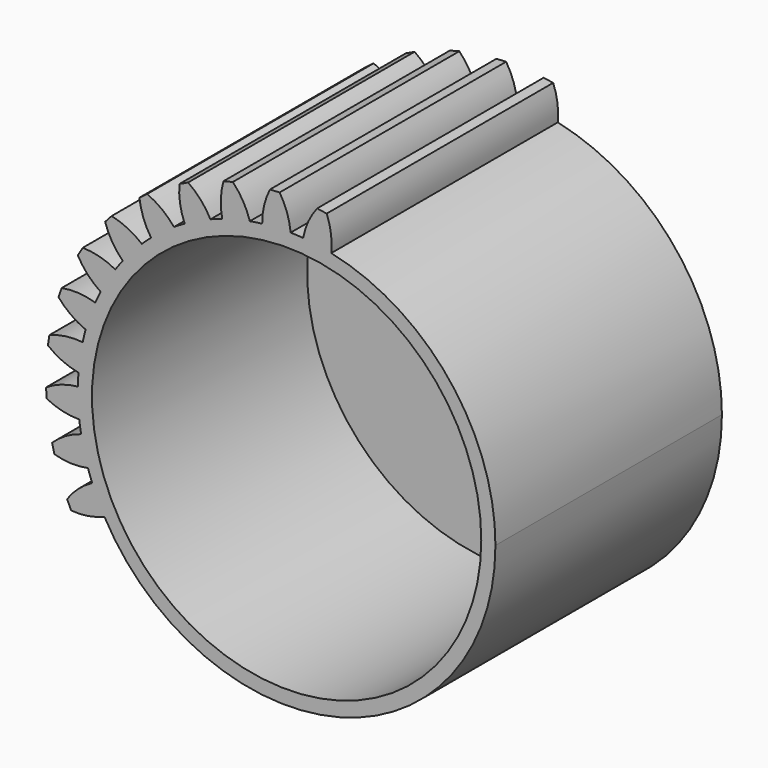
from build123d import *

# Parameters (mm, degrees)
F0_R     = 55
F1_DEPTH = 80
F2_DEPTH = 80
F3_DEPTH = 4


with BuildPart() as f1:
    # F0 (on Front) → F1 (new body)
    with BuildSketch(Plane.XZ):
        with BuildLine():
            ThreePointArc((-51.4911909934, -28.8037714558), (14.8832075069, -57.0919445658), (59, 0))
            ThreePointArc((59, 0), (45.9639360321, 36.9907635016), (12.6163869683, 57.6352910973))
            ThreePointArc((12.6163869683, 57.6352910973), (8.6570979929, 58.3614140879), (4.6575122934, 58.8158786319))
            ThreePointArc((4.6575122934, 58.8158786319), (2.8949927853, 58.9289319161), (1.1298791308, 58.9891801363))
            ThreePointArc((1.1298791308, 58.9891801363), (-2.8949927853, 58.9289319161), (-6.9063892013, 58.5943835892))
            ThreePointArc((-6.9063892013, 58.5943835892), (-8.6570979929, 58.3614140879), (-10.4000493282, 58.0761480642))
            ThreePointArc((-10.4000493282, 58.0761480642), (-14.3358306143, 57.2318439385), (-18.2048820321, 56.1211392454))
            ThreePointArc((-18.2048820321, 56.1211392454), (-19.8765013501, 55.5510998458), (-21.5303097238, 54.9312821914))
            ThreePointArc((-21.5303097238, 54.9312821914), (-25.2257505124, 53.3353682943), (-28.8037714558, 51.4911909934))
            ThreePointArc((-28.8037714558, 51.4911909934), (-30.3320619074, 50.60598799), (-31.8331723911, 49.6754379499))
            ThreePointArc((-31.8331723911, 49.6754379499), (-35.1462589651, 47.3892443574), (-38.2957480959, 44.8824651482))
            ThreePointArc((-38.2957480959, 44.8824651482), (-39.621978336, 43.7161163959), (-40.9127040957, 42.5105944863))
            ThreePointArc((-40.9127040957, 42.5105944863), (-43.7161163959, 39.621978336), (-46.3160406131, 36.5489313377))
            ThreePointArc((-46.3160406131, 36.5489313377), (-47.3892443574, 35.1462589651), (-48.419983526, 33.7120927168))
            ThreePointArc((-48.419983526, 33.7120927168), (-50.60598799, 30.3320619074), (-52.5564336639, 26.8108425927))
            ThreePointArc((-52.5564336639, 26.8108425927), (-53.3353682943, 25.2257505124), (-54.0665101436, 23.6180541301))
            ThreePointArc((-54.0665101436, 23.6180541301), (-55.5510998458, 19.8765013501), (-56.777112443, 16.0424282026))
            ThreePointArc((-56.777112443, 16.0424282026), (-57.2318439385, 14.3358306143), (-57.6352910973, 12.6163869683))
            ThreePointArc((-57.6352910973, 12.6163869683), (-58.3614140879, 8.6570979929), (-58.8158786319, 4.6575122934))
            ThreePointArc((-58.8158786319, 4.6575122934), (-58.9289319161, 2.8949927853), (-58.9891801363, 1.1298791308))
            ThreePointArc((-58.9891801363, 1.1298791308), (-58.9289319161, -2.8949927853), (-58.5943835892, -6.9063892013))
            ThreePointArc((-58.5943835892, -6.9063892013), (-58.3614140879, -8.6570979929), (-58.0761480642, -10.4000493282))
            ThreePointArc((-58.0761480642, -10.4000493282), (-57.2318439385, -14.3358306143), (-56.1211392454, -18.2048820321))
            ThreePointArc((-56.1211392454, -18.2048820321), (-55.5510998458, -19.8765013501), (-54.9312821914, -21.5303097238))
            ThreePointArc((-54.9312821914, -21.5303097238), (-53.3353682943, -25.2257505124), (-51.4911909934, -28.8037714558))
        make_face()
        Circle(F0_R, mode=Mode.SUBTRACT)
    extrude(amount=F1_DEPTH)

    # F0 (on Front) → F2 (join)
    with BuildSketch(Plane.XZ):
        with BuildLine():
            ThreePointArc((-51.4911909934, -28.8037714558), (14.8832075069, -57.0919445658), (59, 0))
            ThreePointArc((59, 0), (45.9639360321, 36.9907635016), (12.6163869683, 57.6352910973))
            ThreePointArc((12.6163869683, 57.6352910973), (8.6570979929, 58.3614140879), (4.6575122934, 58.8158786319))
            ThreePointArc((4.6575122934, 58.8158786319), (2.8949927853, 58.9289319161), (1.1298791308, 58.9891801363))
            ThreePointArc((1.1298791308, 58.9891801363), (-2.8949927853, 58.9289319161), (-6.9063892013, 58.5943835892))
            ThreePointArc((-6.9063892013, 58.5943835892), (-8.6570979929, 58.3614140879), (-10.4000493282, 58.0761480642))
            ThreePointArc((-10.4000493282, 58.0761480642), (-14.3358306143, 57.2318439385), (-18.2048820321, 56.1211392454))
            ThreePointArc((-18.2048820321, 56.1211392454), (-19.8765013501, 55.5510998458), (-21.5303097238, 54.9312821914))
            ThreePointArc((-21.5303097238, 54.9312821914), (-25.2257505124, 53.3353682943), (-28.8037714558, 51.4911909934))
            ThreePointArc((-28.8037714558, 51.4911909934), (-30.3320619074, 50.60598799), (-31.8331723911, 49.6754379499))
            ThreePointArc((-31.8331723911, 49.6754379499), (-35.1462589651, 47.3892443574), (-38.2957480959, 44.8824651482))
            ThreePointArc((-38.2957480959, 44.8824651482), (-39.621978336, 43.7161163959), (-40.9127040957, 42.5105944863))
            ThreePointArc((-40.9127040957, 42.5105944863), (-43.7161163959, 39.621978336), (-46.3160406131, 36.5489313377))
            ThreePointArc((-46.3160406131, 36.5489313377), (-47.3892443574, 35.1462589651), (-48.419983526, 33.7120927168))
            ThreePointArc((-48.419983526, 33.7120927168), (-50.60598799, 30.3320619074), (-52.5564336639, 26.8108425927))
            ThreePointArc((-52.5564336639, 26.8108425927), (-53.3353682943, 25.2257505124), (-54.0665101436, 23.6180541301))
            ThreePointArc((-54.0665101436, 23.6180541301), (-55.5510998458, 19.8765013501), (-56.777112443, 16.0424282026))
            ThreePointArc((-56.777112443, 16.0424282026), (-57.2318439385, 14.3358306143), (-57.6352910973, 12.6163869683))
            ThreePointArc((-57.6352910973, 12.6163869683), (-58.3614140879, 8.6570979929), (-58.8158786319, 4.6575122934))
            ThreePointArc((-58.8158786319, 4.6575122934), (-58.9289319161, 2.8949927853), (-58.9891801363, 1.1298791308))
            ThreePointArc((-58.9891801363, 1.1298791308), (-58.9289319161, -2.8949927853), (-58.5943835892, -6.9063892013))
            ThreePointArc((-58.5943835892, -6.9063892013), (-58.3614140879, -8.6570979929), (-58.0761480642, -10.4000493282))
            ThreePointArc((-58.0761480642, -10.4000493282), (-57.2318439385, -14.3358306143), (-56.1211392454, -18.2048820321))
            ThreePointArc((-56.1211392454, -18.2048820321), (-55.5510998458, -19.8765013501), (-54.9312821914, -21.5303097238))
            ThreePointArc((-54.9312821914, -21.5303097238), (-53.3353682943, -25.2257505124), (-51.4911909934, -28.8037714558))
        make_face()
        Circle(F0_R, mode=Mode.SUBTRACT)
        with BuildLine():
            ThreePointArc((4.6575122934, 58.8158786319), (8.6570979929, 58.3614140879), (12.6163869683, 57.6352910973))
            ThreePointArc((12.6163869683, 57.6352910973), (12.5370476129, 62.4200348178), (11.3233557269, 67.048967655))
            ThreePointArc((11.3233557269, 67.048967655), (9.9744720661, 67.2424287026), (8.627512105, 67.4488582809))
            ThreePointArc((8.627512105, 67.4488582809), (6.1223731095, 63.371561895), (4.6575122934, 58.8158786319))
        make_face()
        with BuildLine():
            ThreePointArc((-60.8748649556, -30.2990637669), (-56.092936255, -30.1167862131), (-51.4911909934, -28.8037714558))
            ThreePointArc((-51.4911909934, -28.8037714558), (-53.3353682943, -25.2257505124), (-54.9312821914, -21.5303097238))
            ThreePointArc((-54.9312821914, -21.5303097238), (-58.8655726136, -24.2545391707), (-62.0400985212, -27.8353843876))
            ThreePointArc((-62.0400985212, -27.8353843876), (-61.4515558937, -29.0644213614), (-60.8748649556, -30.2990637669))
        make_face()
        with BuildLine():
            ThreePointArc((-6.9063892013, 58.5943835892), (-2.8949927853, 58.9289319161), (1.1298791308, 58.9891801363))
            ThreePointArc((1.1298791308, 58.9891801363), (0.1186070656, 63.6665080075), (-1.9748240689, 67.9697176573))
            ThreePointArc((-1.9748240689, 67.9697176573), (-3.3355316865, 67.8963072574), (-4.6968826025, 67.8359914967))
            ThreePointArc((-4.6968826025, 67.8359914967), (-6.3584449898, 63.3483108443), (-6.9063892013, 58.5943835892))
        make_face()
        with BuildLine():
            ThreePointArc((-65.6162256021, -17.8407787457), (-60.8906197339, -18.5949116141), (-56.1211392454, -18.2048820321))
            ThreePointArc((-56.1211392454, -18.2048820321), (-57.2318439385, -14.3358306143), (-58.0761480642, -10.4000493282))
            ThreePointArc((-58.0761480642, -10.4000493282), (-62.4663129991, -12.3043914847), (-66.2784295279, -15.1971124833))
            ThreePointArc((-66.2784295279, -15.1971124833), (-65.940968801, -16.517352827), (-65.6162256021, -17.8407787457))
        make_face()
        with BuildLine():
            ThreePointArc((-18.2048820321, 56.1211392454), (-14.3358306143, 57.2318439385), (-10.4000493282, 58.0761480642))
            ThreePointArc((-10.4000493282, 58.0761480642), (-12.3043914847, 62.4663129991), (-15.1971124833, 66.2784295279))
            ThreePointArc((-15.1971124833, 66.2784295279), (-16.517352827, 65.940968801), (-17.8407787457, 65.6162256021))
            ThreePointArc((-17.8407787457, 65.6162256021), (-18.5949116141, 60.8906197339), (-18.2048820321, 56.1211392454))
        make_face()
        with BuildLine():
            ThreePointArc((-67.8359914967, -4.6968826025), (-63.3483108443, -6.3584449898), (-58.5943835892, -6.9063892013))
            ThreePointArc((-58.5943835892, -6.9063892013), (-58.9289319161, -2.8949927853), (-58.9891801363, 1.1298791308))
            ThreePointArc((-58.9891801363, 1.1298791308), (-63.6665080075, 0.1186070656), (-67.9697176573, -1.9748240689))
            ThreePointArc((-67.9697176573, -1.9748240689), (-67.8963072574, -3.3355316865), (-67.8359914967, -4.6968826025))
        make_face()
        with BuildLine():
            ThreePointArc((-28.8037714558, 51.4911909934), (-25.2257505124, 53.3353682943), (-21.5303097238, 54.9312821914))
            ThreePointArc((-21.5303097238, 54.9312821914), (-24.2545391707, 58.8655726136), (-27.8353843876, 62.0400985212))
            ThreePointArc((-27.8353843876, 62.0400985212), (-29.0644213614, 61.4515558937), (-30.2990637669, 60.8748649556))
            ThreePointArc((-30.2990637669, 60.8748649556), (-30.1167862131, 56.092936255), (-28.8037714558, 51.4911909934))
        make_face()
        with BuildLine():
            ThreePointArc((-67.4488582809, 8.627512105), (-63.371561895, 6.1223731095), (-58.8158786319, 4.6575122934))
            ThreePointArc((-58.8158786319, 4.6575122934), (-58.3614140879, 8.6570979929), (-57.6352910973, 12.6163869683))
            ThreePointArc((-57.6352910973, 12.6163869683), (-62.4200348178, 12.5370476129), (-67.048967655, 11.3233557269))
            ThreePointArc((-67.048967655, 11.3233557269), (-67.2424287026, 9.9744720661), (-67.4488582809, 8.627512105))
        make_face()
        with BuildLine():
            ThreePointArc((-38.2957480959, 44.8824651482), (-35.1462589651, 47.3892443574), (-31.8331723911, 49.6754379499))
            ThreePointArc((-31.8331723911, 49.6754379499), (-35.2725985184, 53.0026612847), (-39.4039580801, 55.4176013207))
            ThreePointArc((-39.4039580801, 55.4176013207), (-40.4945604824, 54.6005941558), (-41.5929727595, 53.7941173879))
            ThreePointArc((-41.5929727595, 53.7941173879), (-40.4812896077, 49.1396326931), (-38.2957480959, 44.8824651482))
        make_face()
        with BuildLine():
            ThreePointArc((-64.4697032671, 21.6203563608), (-60.9594793614, 18.3679118437), (-56.777112443, 16.0424282026))
            ThreePointArc((-56.777112443, 16.0424282026), (-55.5510998458, 19.8765013501), (-54.0665101436, 23.6180541301))
            ThreePointArc((-54.0665101436, 23.6180541301), (-58.7747946957, 24.4736964513), (-63.5515634272, 24.1863853124))
            ThreePointArc((-63.5515634272, 24.1863853124), (-64.0044613228, 22.9011624509), (-64.4697032671, 21.6203563608))
        make_face()
        with BuildLine():
            ThreePointArc((-46.3160406131, 36.5489313377), (-43.7161163959, 39.621978336), (-40.9127040957, 42.5105944863))
            ThreePointArc((-40.9127040957, 42.5105944863), (-44.9351516862, 45.102887407), (-49.4582597616, 46.66543678))
            ThreePointArc((-49.4582597616, 46.66543678), (-50.3685163537, 45.6513622048), (-51.2884871345, 44.6460920571))
            ThreePointArc((-51.2884871345, 44.6460920571), (-49.2901197448, 40.2979206046), (-46.3160406131, 36.5489313377))
        make_face()
        with BuildLine():
            ThreePointArc((-59.0130137119, 33.7823424464), (-56.2047582223, 29.9075820266), (-52.5564336639, 26.8108425927))
            ThreePointArc((-52.5564336639, 26.8108425927), (-50.60598799, 30.3320619074), (-48.419983526, 33.7120927168))
            ThreePointArc((-48.419983526, 33.7120927168), (-52.8708721746, 35.4698348601), (-57.611908257, 36.1199456742))
            ThreePointArc((-57.611908257, 36.1199456742), (-58.3068383884, 34.9477740059), (-59.0130137119, 33.7823424464))
        make_face()
    extrude(amount=F2_DEPTH)


with BuildPart() as f3:
    # F0 (on Front) → F3 (new body)
    with BuildSketch(Plane.XZ):
        Circle(F0_R)
    extrude(amount=F3_DEPTH)


solid = Compound([f1.part, f3.part])
